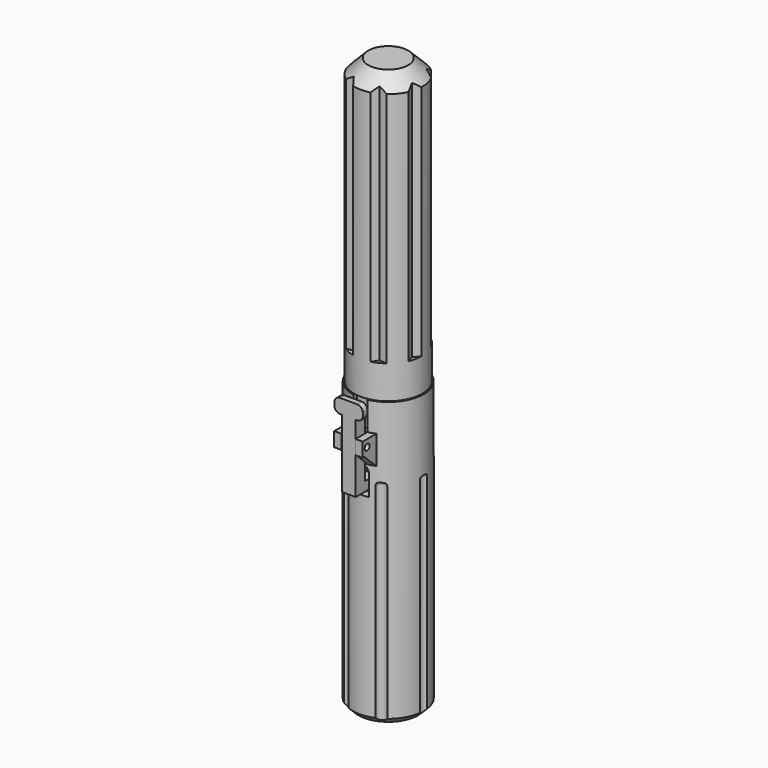
from build123d import *

# Parameters (mm, degrees)
F0_R         = 12.5
F1_DEPTH     = 100
F3_W         = 10
F3_H         = 5
F4_DEPTH     = 17.5
F5_SIZE      = 4.99999
F6_W         = 5
F6_H         = 10
F7_DEPTH     = 5
F8_R         = 1.1
F9_DEPTH     = 25
F11_DEPTH    = 9
F2_R         = 9.7
F12_DEPTH    = 95
F13_SIZE     = 2
F14_R        = 1.8937903908
F15_DEPTH    = 75
F16_R        = 1
F17_R        = 2.9999
F18_R        = 7.9
F19_DEPTH    = 5
F21_DEPTH    = 2
F22_R        = 9.5
F23_DEPTH    = 35
F24_W        = 7
F24_H        = 7
F25_DEPTH    = 25
F26_SIZE     = 2
F27_R        = 2
F28_DEPTH    = 10
F29_R        = 8.5
F29_R_2      = 7.5
F30_DEPTH    = 1
F31_W        = 4
F31_H        = 28
F32_DEPTH    = 4.8
F33_T1_DEPTH = 30.5168298797
F34_W        = 10
F34_H        = 5
F35_DEPTH    = 2
F36_R        = 2
F37_R        = 1.2
F38_DEPTH    = 25
F39_W        = 4.8
F39_H        = 3.2907555205
F40_DEPTH    = 6
F41_SIZE     = 1
F42_R        = 12
F43_DEPTH    = 100
F44_SIZE     = 5
F45_R        = 10
F46_DEPTH    = 93.1
F47_SIZE     = 5
F49_DEPTH    = 88.3
F50_R        = 1.975
F51_DEPTH    = 90
F52_SIZE2    = 1.7632698071
F52_SIZE     = 10


# Not quite as in the source:
# - a fillet or chamfer that OpenCascade refuses, or shapes differently, is made with other operations: its cross-section is extruded or revolved along the edge and cut away or added
# - a fillet or chamfer is up to 0.001 mm smaller than in the source, because OpenCascade refuses the exact size


with BuildPart() as f1:
    # F0 (on Top) → F1 (new body)
    with BuildSketch(Plane.XY):
        Circle(F0_R)
    extrude(amount=F1_DEPTH)

    # F3 (on Front) → F4 (join)
    with BuildSketch(Plane.XZ):
        with Locations((0, 87.5)):
            Rectangle(F3_W, F3_H)
    extrude(amount=F4_DEPTH)

    # F5 (size 5 in the source; OpenCascade refuses exactly that, so slightly less here)
    f5_edges = [f1.edges().sort_by_distance(p)[0] for p in [
        (0, -12.5, 85),
    ]]
    chamfer(f5_edges, length=F5_SIZE)

    # F6 (on face) → F7 (cut)
    with BuildSketch(Plane.XZ.offset(17.5)):
        with Locations((0, 85)):
            Rectangle(F6_W, F6_H)
    extrude(amount=-F7_DEPTH, mode=Mode.SUBTRACT)

    # F8 (on face) → F9 (cut)
    with BuildSketch(Plane.YZ.offset(5)):
        with Locations((-15.5, 87.5)):
            Circle(F8_R)
    extrude(amount=-F9_DEPTH, mode=Mode.SUBTRACT)

    # F10 (on face) → F11 (cut)
    with BuildSketch(Plane.XZ.offset(12.5)):
        Polygon((0, 80), (-3, 80), (-3, 70), (3, 70), (3, 80), align=None)
    extrude(amount=-F11_DEPTH, mode=Mode.SUBTRACT)

    # F2 (on face) → F12 (cut)
    with BuildSketch(Plane.XY.offset(100)):
        Circle(F2_R)
    extrude(amount=-F12_DEPTH, mode=Mode.SUBTRACT)

    # F13
    f13_edges = [f1.edges().sort_by_distance(p)[0] for p in [
        (-12.5, 0, 0),
    ]]
    chamfer(f13_edges, length=F13_SIZE)

    # F14 (on face) → F15 (cut)
    with BuildSketch(Plane(origin=(0, 0, 0), x_dir=(1, 0, 0), z_dir=(0, 0, -1))):
        with Locations((13.3886011317, 0)):
            Circle(F14_R)
        with Locations((6.6943005659, 11.5948687012)):
            Circle(F14_R)
        with Locations((-6.6943005659, 11.5948687012)):
            Circle(F14_R)
        with Locations((-13.3886011317, 0)):
            Circle(F14_R)
        with Locations((-6.6943005659, -11.5948687012)):
            Circle(F14_R)
        with Locations((6.6943005659, -11.5948687012)):
            Circle(F14_R)
    extrude(amount=-F15_DEPTH, mode=Mode.SUBTRACT)

    # F16
    f16_edges = [f1.edges().sort_by_distance(p)[0] for p in [
        (-5.747405, 9.954798, 75),
        (5.747405, 9.954798, 75),
        (11.494811, 0, 75),
        (5.747405, -9.954798, 75),
        (-5.747405, -9.954798, 75),
        (-11.494811, 0, 75),
    ]]
    fillet(f16_edges, radius=F16_R)

    # F17 (radius 3 in the source; OpenCascade refuses exactly that, so slightly less here)
    f17_edges = [f1.edges().sort_by_distance(p)[0] for p in [
        (-3, -10.679543, 80),
        (3, -10.679543, 80),
    ]]
    fillet(f17_edges, radius=F17_R)

    # F18 (on face) → F19 (join)
    with BuildSketch(Plane.XY.offset(5)):
        Circle(F18_R)
    extrude(amount=F19_DEPTH)

    # F20 (on face) → F21 (cut)
    with BuildSketch(Plane.XZ.offset(12.5)):
        Polygon((0, 90), (2.5, 90), (2.5, 101.5290468931), (-2.5, 101.5290468931), (-2.5, 90), align=None)
    extrude(amount=-F21_DEPTH, mode=Mode.SUBTRACT)


with BuildPart() as f23:
    # F22 (on face) → F23 (new body)
    with BuildSketch(Plane.XY.offset(100)):
        Circle(F22_R)
    extrude(amount=-F23_DEPTH)

    # F24 (on face) → F25 (cut)
    with BuildSketch(Plane.XZ.offset(12.5)):
        with Locations((0, 73)):
            Rectangle(F24_W, F24_H)
    extrude(amount=-F25_DEPTH, mode=Mode.SUBTRACT)

    # F26
    f26_edges = [f23.edges().sort_by_distance(p)[0] for p in [
        (-3.5, 0, 76.5),
        (3.5, 0, 76.5),
    ]]
    chamfer(f26_edges, length=F26_SIZE)

    # F27 (on face) → F28 (cut)
    with BuildSketch(Plane.XY.offset(100)):
        Circle(F27_R)
    extrude(amount=-F28_DEPTH, mode=Mode.SUBTRACT)

    # F29 (on face) → F30 (cut)
    with BuildSketch(Plane.XY.offset(100)):
        Circle(F29_R)
        Circle(F29_R_2, mode=Mode.SUBTRACT)
    extrude(amount=-F30_DEPTH, mode=Mode.SUBTRACT)


with BuildPart() as f32:
    # F31 (on face) → F32 (new body)
    with BuildSketch(Plane(origin=(2.5, 0, 0), x_dir=(0, -1, 0), z_dir=(-1, 0, 0))):
        with Locations((15.4265365556, 85.999820103)):
            Rectangle(F31_W, F31_H)
    extrude(amount=F32_DEPTH)

    # F33: chamfer of 5 on 1 edges, made by hand

    # F33_s2 → F33_t1 (cut)
    with BuildSketch(Plane.YZ.offset(-15.1584149398)):
        Polygon((-18.4265365556, 99.999820103), (-13.4265365556, 94.999820103), (-13.4265365556, 99.999820103), align=None)
    extrude(amount=F33_T1_DEPTH, mode=Mode.SUBTRACT)

    # F34 (on face) → F35 (join)
    with BuildSketch(Plane.XZ.offset(17.4265365556)):
        with Locations((0, 98.3922585351)):
            Rectangle(F34_W, F34_H)
    extrude(amount=-F35_DEPTH)

    # F36
    f36_edges = [f32.edges().sort_by_distance(p)[0] for p in [
        (-5, -16.426537, 95.892259),
        (-5, -16.426537, 100.892259),
        (5, -16.426537, 95.892259),
        (5, -16.426537, 100.892259),
    ]]
    fillet(f36_edges, radius=F36_R)

    # F37 (on face) → F38 (cut)
    with BuildSketch(Plane(origin=(-2.3, 0, 0), x_dir=(0, -1, 0), z_dir=(-1, 0, 0))):
        with Locations((15.5, 87.5)):
            Circle(F37_R)
    extrude(amount=-F38_DEPTH, mode=Mode.SUBTRACT)

    # F39 (on face) → F40 (join)
    with BuildSketch(Plane(origin=(0, -13.4265365556, 0), x_dir=(-1, 0, 0), z_dir=(0, 1, 0))):
        with Locations((-0.1, 73.6451978633)):
            Rectangle(F39_W, F39_H)
    extrude(amount=F40_DEPTH)

    # F41
    f41_edges = [f32.edges().sort_by_distance(p)[0] for p in [
        (0.1, -7.426537, 75.290576),
    ]]
    chamfer(f41_edges, length=F41_SIZE)


with BuildPart() as f43:
    # F42 (on face) → F43 (new body)
    with BuildSketch(Plane.XY.offset(100)):
        Circle(F42_R)
    extrude(amount=F43_DEPTH)

    # F44
    f44_edges = [f43.edges().sort_by_distance(p)[0] for p in [
        (-12, 0, 200),
    ]]
    chamfer(f44_edges, length=F44_SIZE)

    # F45 (on face) → F46 (cut)
    with BuildSketch(Plane(origin=(0, 0, 100), x_dir=(1, 0, 0), z_dir=(0, 0, -1))):
        Circle(F45_R)
    extrude(amount=-F46_DEPTH, mode=Mode.SUBTRACT)

    # F47
    f47_edges = [f43.edges().sort_by_distance(p)[0] for p in [
        (-10, 0, 193.1),
    ]]
    chamfer(f47_edges, length=F47_SIZE)

    # F48 (on face) → F49 (cut)
    with BuildSketch(Plane.XY.offset(200)):
        Polygon((2.7134206576, 15.2147837694), (-0.0219526665, 16.7687035386), (-2.7353733242, 15.1767606356), (-2.7134206576, 12.0308979635), (0.0219526665, 10.4769781943), (2.7353733242, 12.0689210973), align=None)
        Polygon((-7.7303851014, 9.6634502047), (-10.2036068417, 11.607700213), (-13.1239876104, 10.4379523609), (-13.5711466387, 7.3239545004), (-11.0979248984, 5.3797044921), (-8.1775441297, 6.5494523443), align=None)
        Polygon((-12.3750058745, -0.0187957904), (-15.4371102736, -0.7402183577), (-16.343392203, -3.75278984), (-14.1875697334, -6.043938755), (-11.1254653342, -5.3225161878), (-10.2191834048, -2.3099447055), align=None)
        Polygon((-7.70099482, -9.686888172), (-9.0461548098, -12.5307374074), (-7.2558891224, -15.1176047484), (-4.1204634451, -14.8606228541), (-2.7753034553, -12.0167736187), (-4.5655691427, -9.4299062777), align=None)
        Polygon((2.7720224056, -12.0605561836), (4.1567397337, -14.8853556089), (7.2954464606, -15.0985549383), (9.0494358594, -12.4869548425), (7.6647185314, -9.6621554173), (4.5260118045, -9.4489560878), align=None)
        Polygon((11.1576502208, -5.3523793984), (14.2295244757, -6.0309974309), (16.3531620587, -3.7099853053), (15.404925387, -0.7103551471), (12.3330511322, -0.0317371145), (10.2094135491, -2.3527492402), align=None)
        Polygon((11.1413398452, 5.3862482424), (13.5871870581, 7.3648248224), (13.0966130829, 10.4722789325), (10.1601918949, 11.6011564627), (7.714344682, 9.6225798827), (8.2049186571, 6.5151257726), align=None)
    extrude(amount=-F49_DEPTH, mode=Mode.SUBTRACT)


with BuildPart() as f51:
    # F50 (on face) → F51 (new body)
    with BuildSketch(Plane.XY.offset(90)):
        Circle(F50_R)
    extrude(amount=F51_DEPTH)

    # F52
    f52_edges = [f51.edges().sort_by_distance(p)[0] for p in [
        (-1.975, 0, 180),
    ]]
    f52_side = f51.faces().sort_by_distance((-1.975, 0, 135))[0]
    chamfer(f52_edges, length=F52_SIZE, length2=F52_SIZE2, reference=f52_side)


solid = Compound([f1.part, f23.part, f32.part, f43.part, f51.part])
